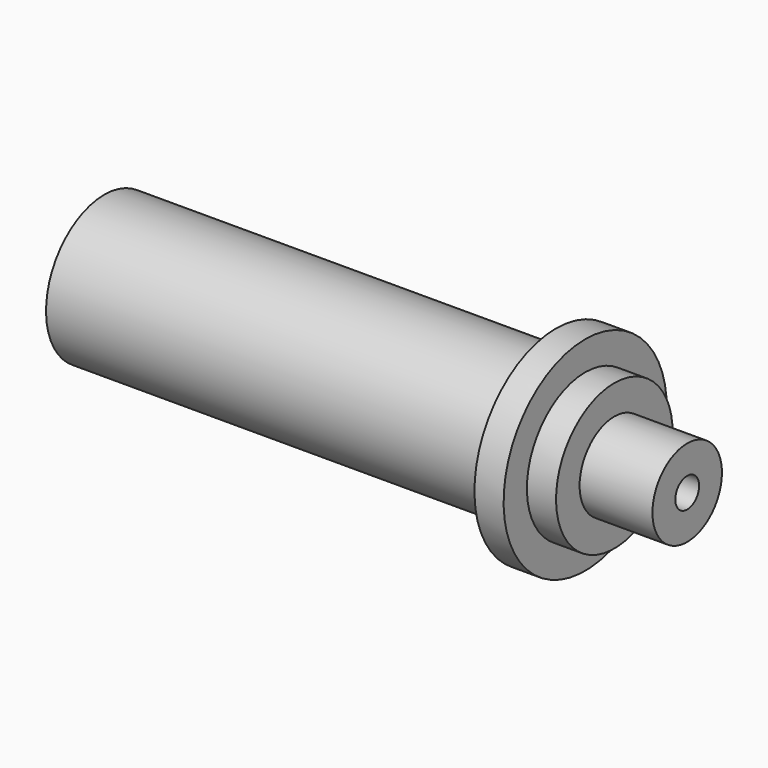
from build123d import *

# Parameters (mm, degrees)
F0_W   = 2.54
F0_H   = 6.35
F0_H_2 = 2.54
F0_W_2 = 39.37
F0_W_3 = 6.35
F0_H_3 = 2.4892


# Not quite as in the source:
# - a feature names something its author has since deleted; it is built from what else it names


with BuildPart() as f1:
    # F0 (on Front) → F1 (revolve)
    with BuildSketch(Plane.XZ):
        Polygon((-23.0985377062, 28.9715196595), (-25.6385377062, 28.9715196595), (-25.6385377062, 22.6215196595), (-23.0985377062, 22.6215196595), (-23.0985377062, 23.9169196595), (-23.0985377062, 26.4061196595), align=None)
        with Locations((-26.9085377062, 25.7965196595)):
            Rectangle(F0_W, F0_H)
        with Locations((-26.9085377062, 30.2415196595)):
            Rectangle(F0_W, F0_H_2)
        with Locations((-47.8635377062, 25.7965196595)):
            Rectangle(F0_W_2, F0_H)
        with Locations((-19.9235377062, 25.1615196595)):
            Rectangle(F0_W_3, F0_H_3)
    revolve(axis=Axis((-42.1485377062, 0, 22.6215196595), (1, 0, 0)))


solid = f1.part
